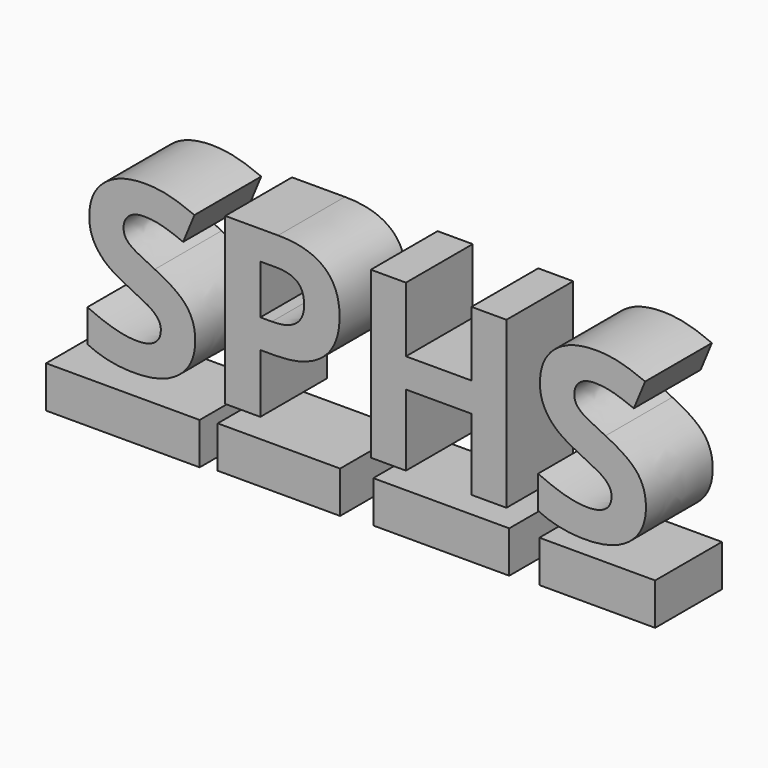
from build123d import *

# Parameters (mm, degrees)
F0_TEXT_SIZE = 35.2777777778
F1_DEPTH     = 12.7
F2_W         = 23.368
F2_H         = 6.35
F6_DEPTH     = 12.7
F3_W         = 18.626666394
F3_H         = 6.35
F7_DEPTH     = 12.7
F4_W         = 20.6887125885
F4_H         = 6.35
F8_DEPTH     = 12.7
F5_W         = 17.6161308197
F5_H         = 6.35
F9_DEPTH     = 12.7


# Not quite as in the source:
# - Text() gives the source's letters only with a copy of the font that has no kerning and outlines rounded to 1/6400 em; it was checked with that copy


with BuildPart() as f1:
    # F0 (on Front) → F1 (new body)
    with BuildSketch(Plane.XZ):
        with Locations((-30.2846139177, -8.5480760674)):
            Text('SPHS', F0_TEXT_SIZE, font='Open Sans', font_style=FontStyle.BOLD, text_align=(TextAlign.LEFT, TextAlign.BOTTOM))
    extrude(amount=F1_DEPTH)


with BuildPart() as f6:
    # F2 (on Front) → F6 (new body)
    with BuildSketch(Plane.XZ):
        with Locations((-23.2601282451, -15.1405424893)):
            Rectangle(F2_W, F2_H)
    extrude(amount=F6_DEPTH)


with BuildPart() as f7:
    # F3 (on Front) → F7 (new body)
    with BuildSketch(Plane.XZ):
        with Locations((0.4819878377, -14.7006325424)):
            Rectangle(F3_W, F3_H)
    extrude(amount=F7_DEPTH)


with BuildPart() as f8:
    # F4 (on Front) → F8 (new body)
    with BuildSketch(Plane.XZ):
        with Locations((25.1838704571, -14.3391415477)):
            Rectangle(F4_W, F4_H)
    extrude(amount=F8_DEPTH)


with BuildPart() as f9:
    # F5 (on Front) → F9 (new body)
    with BuildSketch(Plane.XZ):
        with Locations((48.9217769355, -14.0981483273)):
            Rectangle(F5_W, F5_H)
    extrude(amount=F9_DEPTH)


solid = Compound([f1.part, f6.part, f7.part, f8.part, f9.part])
